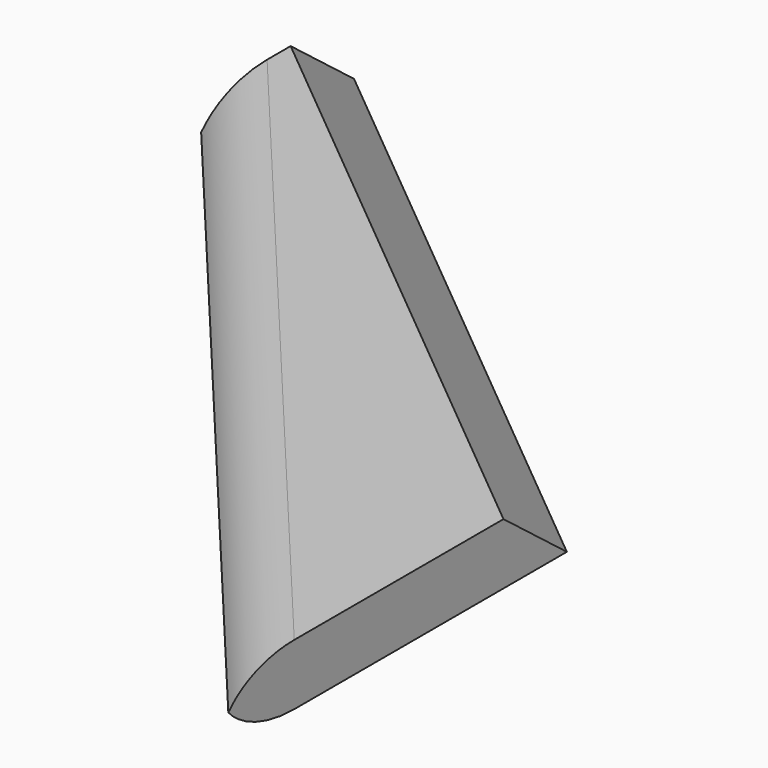
from build123d import *

# Parameters (mm, degrees)
F1_DEPTH    = 5.08
F2_T1_DEPTH = 107.0884939123
F3_SIZE     = 5.07999


# Not quite as in the source:
# - a fillet or chamfer that OpenCascade refuses, or shapes differently, is made with other operations: its cross-section is extruded or revolved along the edge and cut away or added
# - a fillet or chamfer is up to 0.001 mm smaller than in the source, because OpenCascade refuses the exact size


with BuildPart() as f1:
    # F0 (on Top) → F1 (new body)
    with BuildSketch(Plane.XY):
        Polygon((-52.3975975811, 62.6697838306), (0, 0), (0, 36.2825095654), (-52.3975975811, 79.6330347657), align=None)
    extrude(amount=F1_DEPTH)

    # F2: fillet of radius 5.08 on 2 edges, made by hand

    # F2_s2 → F2_t1 (cut)
    with BuildSketch(Plane(origin=(-60.5437814243, 72.412970619, 0), x_dir=(0, 0, 1), z_dir=(0.6414317987, -0.7671800621, 0))):
        with BuildLine():
            ThreePointArc((0, 0), (3.5921024484, -1.4878975516), (5.08, -5.08))
            Line((5.08, -5.08), (5.08, 0))
            Line((5.08, 0), (0, 0))
        make_face()
        with BuildLine():
            ThreePointArc((5.08, 0), (1.4878975516, -1.4878975516), (0, -5.08))
            Line((0, -5.08), (0, 0))
            Line((0, 0), (5.08, 0))
        make_face()
    extrude(amount=F2_T1_DEPTH, mode=Mode.SUBTRACT)

    # F3 (size 5.08 in the source; OpenCascade refuses exactly that, so slightly less here)
    f3_edges = [f1.edges().sort_by_distance(p)[0] for p in [
        (-26.198799, 57.957772, 5.08),
    ]]
    chamfer(f3_edges, length=F3_SIZE)


solid = f1.part
